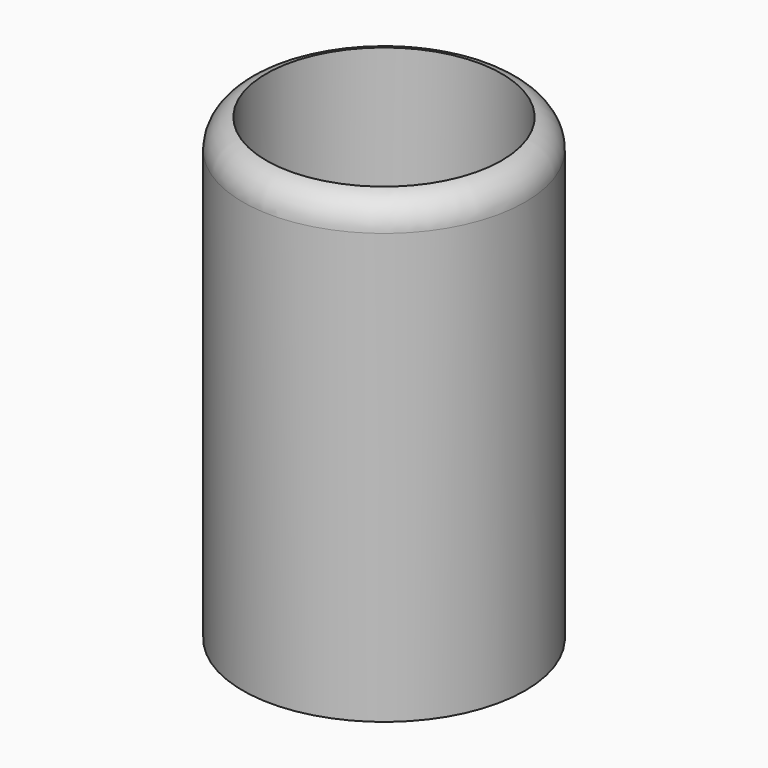
from build123d import *

# Parameters (mm, degrees)
F0_R     = 38.1
F1_DEPTH = 123.825
F2_T     = -6.35


# Not quite as in the source:
# - a fillet or chamfer that OpenCascade refuses, or shapes differently, is made with other operations: its cross-section is extruded or revolved along the edge and cut away or added


with BuildPart() as f1:
    # F0 (on Top) → F1 (new body)
    with BuildSketch(Plane.XY):
        Circle(F0_R)
    extrude(amount=F1_DEPTH)

    # F2
    f2_openings = [f1.faces().sort_by_distance(p)[0] for p in [
        (0, 0, 123.825),
    ]]
    offset(amount=F2_T, openings=f2_openings)

    # F3: fillet of radius 7.971733183 on 1 edges, made by hand

    # F3_s1 → F3_t2 (revolve, cut)
    with BuildSketch(Plane.XZ):
        with BuildLine():
            ThreePointArc((38.1, 116.019968839), (36.3119774413, 121.0508984605), (31.75, 123.825))
            Line((31.75, 123.825), (38.1, 123.825))
            Line((38.1, 123.825), (38.1, 116.019968839))
        make_face()
    revolve(axis=Axis((0, 0, 123.825), (0, 0, 1)), mode=Mode.SUBTRACT)


solid = f1.part
